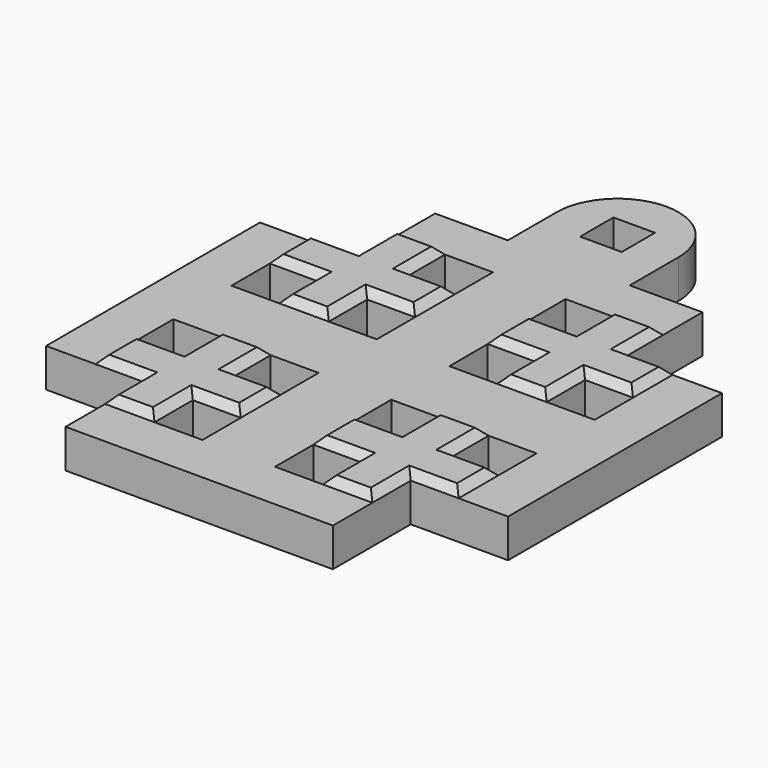
from build123d import *

# Parameters (mm, degrees)
F1_DEPTH  = 6.35
F2_W      = 7.9056663411
F2_H      = 7.9056663411
F3_DEPTH  = 25.4
F4_W      = 6.858
F4_H      = 6.858
F5_DEPTH  = 25.4
F6_W      = 7.9056663411
F6_H      = 8.1499283314
F6_W_2    = 8.1499283314
F6_H_2    = 7.9056663411
F7_DEPTH  = 1.27
F8_SIZE   = 1.26999
F10_DEPTH = 6.35


# Not quite as in the source:
# - a fillet or chamfer is up to 0.001 mm smaller than in the source, because OpenCascade refuses the exact size
# - a feature names something its author has since deleted; it is built from what else it names


with BuildPart() as f1:
    # F0 (on Top) → F1 (new body)
    with BuildSketch(Plane.XY):
        with BuildLine():
            ThreePointArc((13.6716806904, 59.1812469065), (-3.4947036843, 66.2917961397), (3.6158455206, 49.1254117533))
            ThreePointArc((3.6158455206, 49.1254117533), (10.7263947587, 52.0706976733), (13.6716806904, 59.1812469065))
        make_face()
    extrude(amount=F1_DEPTH)

    # F4 (on face) → F5 (cut)
    with BuildSketch(Plane.XY.offset(6.35)):
        with Locations((3.6158455372, 59.1812469065)):
            Rectangle(F4_W, F4_H)
    extrude(amount=-F5_DEPTH, mode=Mode.SUBTRACT)



with BuildPart() as f1b:
    # F0 (on Top) → F1, piece 2 (new body)
    with BuildSketch(Plane.XY):
        Polygon((3.6158455206, 49.1254117533), (-34.4841544628, 49.1254117533), (-34.4841544628, -27.0745882467), (41.7158455372, -27.0745882467), (41.7158455372, 49.1254117533), align=None)
    extrude(amount=F1_DEPTH)

    # F2 (on face) → F3 (cut)
    with BuildSketch(Plane.XY.offset(6.35)):
        Polygon((-34.4841544628, 33.0698170808), (-26.3342261314, 33.0698170808), (-18.4285597903, 33.0698170808), (-18.4285597903, 40.9754834219), (-18.4285597903, 49.1254117533), (-34.4841544628, 49.1254117533), align=None)
        Polygon((25.6602508647, 40.9754834219), (25.6602508647, 33.0698170808), (33.5659172058, 33.0698170808), (41.7158455372, 33.0698170808), (41.7158455372, 49.1254117533), (25.6602508647, 49.1254117533), align=None)
        Polygon((33.5659172058, -11.0189935742), (25.6602508647, -11.0189935742), (25.6602508647, -18.9246599153), (25.6602508647, -27.0745882467), (41.7158455372, -27.0745882467), (41.7158455372, -11.0189935742), align=None)
        Polygon((-18.4285597903, -18.9246599153), (-18.4285597903, -11.0189935742), (-26.3342261314, -11.0189935742), (-34.4841544628, -11.0189935742), (-34.4841544628, -27.0745882467), (-18.4285597903, -27.0745882467), align=None)
        with Locations((-22.3813929609, 1.0837679277)):
            Rectangle(F2_W, F2_H)
        with Locations((-22.3813929609, 20.9670555789)):
            Rectangle(F2_W, F2_H)
        with Locations((-6.3257982884, 37.0226502514)):
            Rectangle(F2_W, F2_H)
        with Locations((-6.3257982884, 20.9670555789)):
            Rectangle(F2_W, F2_H)
        with Locations((-6.3257982884, 1.0837679277)):
            Rectangle(F2_W, F2_H)
        with Locations((-6.3257982884, -14.9718267448)):
            Rectangle(F2_W, F2_H)
        with Locations((13.5574893628, -14.9718267448)):
            Rectangle(F2_W, F2_H)
        with Locations((13.5574893628, 1.0837679277)):
            Rectangle(F2_W, F2_H)
        with Locations((29.6130840353, 1.0837679277)):
            Rectangle(F2_W, F2_H)
        with Locations((29.6130840353, 20.9670555789)):
            Rectangle(F2_W, F2_H)
        with Locations((13.5574893628, 20.9670555789)):
            Rectangle(F2_W, F2_H)
        with Locations((13.5574893628, 37.0226502514)):
            Rectangle(F2_W, F2_H)
    extrude(amount=-F3_DEPTH, mode=Mode.SUBTRACT)

    # F6 (on face) → F7 (join, symmetric)
    with BuildSketch(Plane.XY.offset(6.35)):
        with Locations((-22.3813929609, 28.9948529151)):
            Rectangle(F6_W, F6_H)
        with Locations((-14.3535956246, 28.9948529151)):
            Rectangle(F6_W_2, F6_H)
        with Locations((-14.3535956246, 37.0226502514)):
            Rectangle(F6_W_2, F6_H_2)
        with Locations((-6.3257982884, 28.9948529151)):
            Rectangle(F6_W, F6_H)
        with Locations((-14.3535956246, 20.9670555789)):
            Rectangle(F6_W_2, F6_H_2)
        with Locations((13.5574893628, 28.9948529151)):
            Rectangle(F6_W, F6_H)
        with Locations((29.6130840353, 28.9948529151)):
            Rectangle(F6_W, F6_H)
        with Locations((21.585286699, 28.9948529151)):
            Rectangle(F6_W_2, F6_H)
        with Locations((21.585286699, 37.0226502514)):
            Rectangle(F6_W_2, F6_H_2)
        with Locations((21.585286699, 20.9670555789)):
            Rectangle(F6_W_2, F6_H_2)
        with Locations((-14.3535956246, 1.0837679277)):
            Rectangle(F6_W_2, F6_H_2)
        with Locations((-14.3535956246, -6.9440294085)):
            Rectangle(F6_W_2, F6_H)
        with Locations((-14.3535956246, -14.9718267448)):
            Rectangle(F6_W_2, F6_H_2)
        with Locations((-22.3813929609, -6.9440294085)):
            Rectangle(F6_W, F6_H)
        with Locations((-6.3257982884, -6.9440294085)):
            Rectangle(F6_W, F6_H)
        with Locations((13.5574893628, -6.9440294085)):
            Rectangle(F6_W, F6_H)
        with Locations((21.585286699, -6.9440294085)):
            Rectangle(F6_W_2, F6_H)
        with Locations((29.6130840353, -6.9440294085)):
            Rectangle(F6_W, F6_H)
        with Locations((21.585286699, -14.9718267448)):
            Rectangle(F6_W_2, F6_H_2)
        with Locations((21.585286699, 1.0837679277)):
            Rectangle(F6_W_2, F6_H_2)
    extrude(amount=F7_DEPTH, both=True)

    # F8 (size 1.27 in the source; OpenCascade refuses exactly that, so slightly less here)
    f8_edges = [f1b.edges().sort_by_distance(p)[0] for p in [
        (-22.381393, 33.069817, 7.62),
        (-18.42856, 37.02265, 7.62),
        (-14.353596, 40.975483, 7.62),
        (-10.278631, 37.02265, 7.62),
        (-6.325798, 33.069817, 7.62),
        (-2.372965, 28.994853, 7.62),
        (-6.325798, 24.919889, 7.62),
        (-10.278631, 20.967056, 7.62),
        (-14.353596, 17.014222, 7.62),
        (-18.42856, 20.967056, 7.62),
        (-22.381393, 24.919889, 7.62),
        (-26.334226, 28.994853, 7.62),
        (-10.278631, 1.083768, 7.62),
        (-6.325798, -2.869065, 7.62),
        (-2.372965, -6.944029, 7.62),
        (-6.325798, -11.018994, 7.62),
        (-14.353596, -18.92466, 7.62),
        (-26.334226, -6.944029, 7.62),
        (-22.381393, -11.018994, 7.62),
        (-18.42856, -14.971827, 7.62),
        (-22.381393, -2.869065, 7.62),
        (-18.42856, 1.083768, 7.62),
        (-14.353596, 5.036601, 7.62),
        (-10.278631, -14.971827, 7.62),
        (25.660251, 1.083768, 7.62),
        (25.660251, -14.971827, 7.62),
        (21.585287, -18.92466, 7.62),
        (17.510323, -14.971827, 7.62),
        (13.557489, -11.018994, 7.62),
        (9.604656, -6.944029, 7.62),
        (13.557489, -2.869065, 7.62),
        (17.510323, 1.083768, 7.62),
        (21.585287, 5.036601, 7.62),
        (29.613084, -2.869065, 7.62),
        (29.613084, -11.018994, 7.62),
        (33.565917, -6.944029, 7.62),
        (29.613084, 33.069817, 7.62),
        (25.660251, 37.02265, 7.62),
        (21.585287, 40.975483, 7.62),
        (17.510323, 37.02265, 7.62),
        (13.557489, 33.069817, 7.62),
        (9.604656, 28.994853, 7.62),
        (17.510323, 20.967056, 7.62),
        (13.557489, 24.919889, 7.62),
        (21.585287, 17.014222, 7.62),
        (29.613084, 24.919889, 7.62),
        (33.565917, 28.994853, 7.62),
        (25.660251, 20.967056, 7.62),
    ]]
    chamfer(f8_edges, length=F8_SIZE)


with BuildPart() as f1_1:
    add(f1.part)

    add(f1b.part)  # F10 merges F1b
    # F9 (on face) → F10 (join)
    with BuildSketch(Plane.XY.offset(6.35)):
        with BuildLine():
            Line((-6.439989616, 49.1254117533), (3.6158455372, 49.1254117533))
            ThreePointArc((3.6158455372, 49.1254117533), (-3.4947036902, 52.0706976792), (-6.439989616, 59.1812469065))
            Line((-6.439989616, 59.1812469065), (-6.439989616, 49.1254117533))
        make_face()
        with BuildLine():
            Line((3.6158455372, 49.1254117533), (13.6716806904, 49.1254117533))
            Line((13.6716806904, 49.1254117533), (13.6716806904, 59.1812469065))
            ThreePointArc((13.6716806904, 59.1812469065), (10.7263947645, 52.0706976792), (3.6158455372, 49.1254117533))
        make_face()
    extrude(amount=-F10_DEPTH)


solid = f1_1.part
